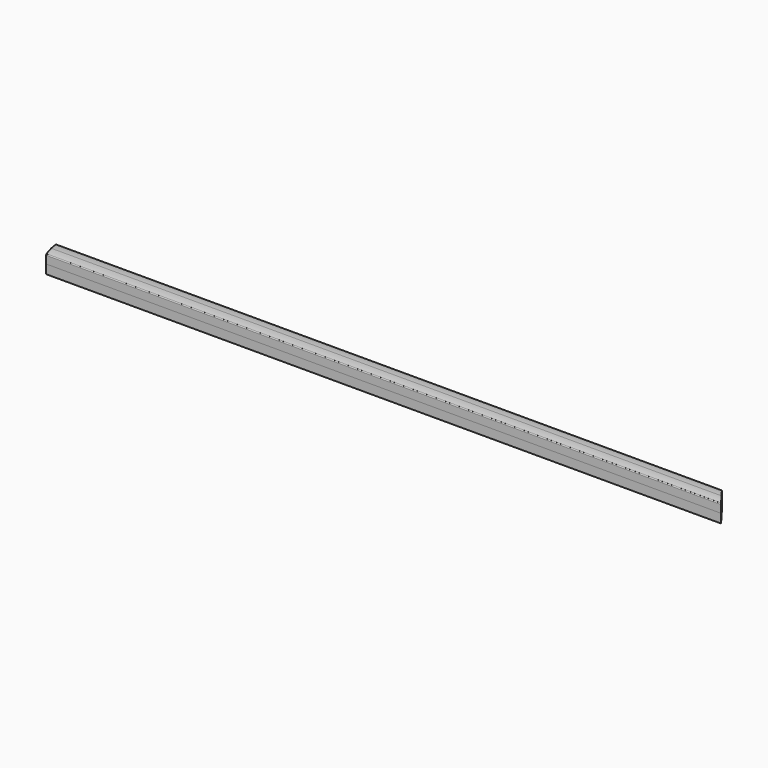
from build123d import *

# Parameters (mm, degrees)
F2_DEPTH      = 1000
F4_DEPTH      = 1000
F8_DEPTH      = 10.001
F8_DEPTH_BACK = 10.001


with BuildPart() as f2:
    # F1 (on Right) → F2 (new body)
    with BuildSketch(Plane.YZ):
        with BuildLine():
            Line((0, -9), (0, -10))
            Line((0, -10), (10, -10))
            Line((10, -10), (10, -0.2))
            Line((10, -0.2), (9, -0.2))
            ThreePointArc((9, -0.2), (8.5, -0.7), (9, -1.2))
            ThreePointArc((9, -1.2), (9.5, -1.7), (9, -2.2))
            Line((9, -2.2), (9, -9))
            Line((9, -9), (0, -9))
        make_face()
    extrude(amount=F2_DEPTH)

    # F5: F2 across plane


with BuildPart() as f4:
    # F3 (on Right) → F4 (new body)
    with BuildSketch(Plane.YZ):
        with BuildLine():
            Line((9, -0.2), (10, -0.2))
            Line((10, -0.2), (10, 8.1663783152))
            ThreePointArc((10, 8.1663783152), (9.7693092582, 8.8052548802), (9.1836734694, 9.1493656277))
            ThreePointArc((9.1836734694, 9.1493656277), (4.6114920912, 9.7868872364), (0, 10))
            Line((0, 10), (0, 9))
            ThreePointArc((0, 9), (4.5192622493, 8.7911494917), (9, 8.1663783152))
            Line((9, 8.1663783152), (9, 0.8))
            ThreePointArc((9, 0.8), (7.5, -0.7), (9, -2.2))
            ThreePointArc((9, -2.2), (9.5, -1.7), (9, -1.2))
            ThreePointArc((9, -1.2), (8.5, -0.7), (9, -0.2))
        make_face()
    extrude(amount=F4_DEPTH)

    # F6: F4 across plane


with BuildPart() as f2_1:
    add(f2.part)
    add(f2.part.mirror(Plane.XZ))


with BuildPart() as f4_1:
    add(f4.part)
    add(f4.part.mirror(Plane.XZ))


with BuildPart() as f8_tool:
    # F7 (on Top) → F8 (new body, two sides)
    with BuildSketch(Plane.XY) as f8_sk:
        Polygon((0, 10), (0, 0), (0, -10), (4.8015751816, -10), align=None)
        Polygon((739.8015751816, 10), (724.7304941795, 10), (739.8015751816, -10), (1016.9613361359, -10), (1016.9613361359, 10), align=None)
    extrude(amount=F8_DEPTH)
    extrude(f8_sk.sketch, amount=-F8_DEPTH_BACK)


with BuildPart() as f2_2:
    add(f2_1.part)

    # F8: cut by f8_tool
    add(f8_tool.part, mode=Mode.SUBTRACT)


with BuildPart() as f4_2:
    add(f4_1.part)

    # F8: cut by f8_tool
    add(f8_tool.part, mode=Mode.SUBTRACT)


solid = Compound([f2_2.part, f4_2.part])
